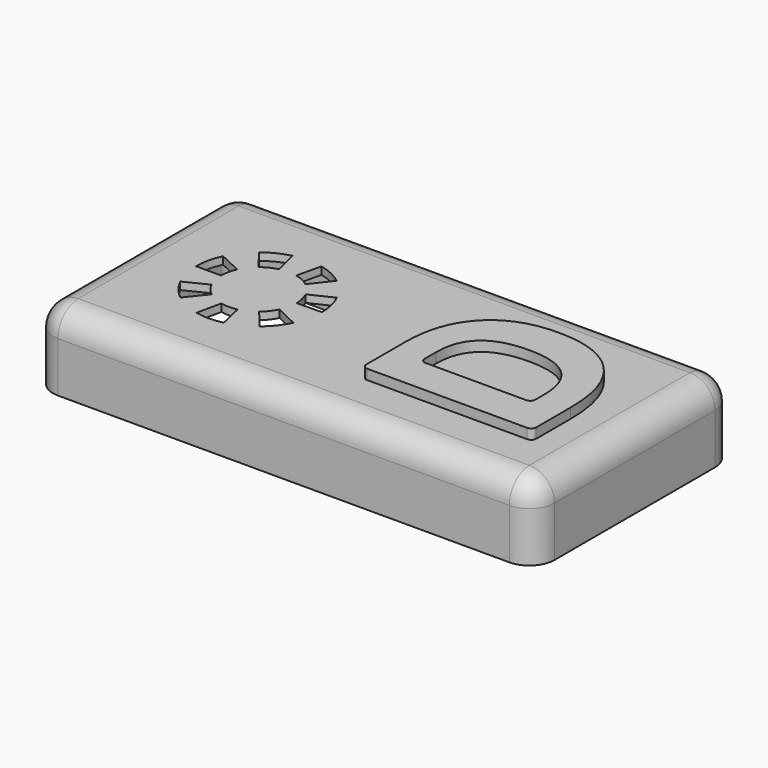
from build123d import *

# Parameters (mm, degrees)
F1_DEPTH     = 15
F2_R         = 5
F3_T         = -1.5
F5_DEPTH     = 1.5
F6_TEXT_SIZE = 47.5117315849
F7_DEPTH     = 2
F8_R         = 1


# Not quite as in the source:
# - Text() gives the source's letters only with a copy of the font that has no kerning and outlines rounded to 1/6400 em; it was checked with that copy


with BuildPart() as f1:
    # F0 (on Top) → F1 (new body)
    with BuildSketch(Plane.XY):
        with BuildLine():
            Line((45, 25), (-45, 25))
            ThreePointArc((-45, 25), (-48.5355339059, 23.5355339059), (-50, 20))
            Line((-50, 20), (-50, -20))
            ThreePointArc((-50, -20), (-48.5355339059, -23.5355339059), (-45, -25))
            Line((-45, -25), (45, -25))
            ThreePointArc((45, -25), (48.5355339059, -23.5355339059), (50, -20))
            Line((50, -20), (50, 20))
            ThreePointArc((50, 20), (48.5355339059, 23.5355339059), (45, 25))
        make_face()
    extrude(amount=F1_DEPTH)

    # F2
    f2_edges = [f1.edges().sort_by_distance(p)[0] for p in [
        (0, -25, 15),
    ]]
    fillet(f2_edges, radius=F2_R)

    # F3
    f3_openings = [f1.faces().sort_by_distance(p)[0] for p in [
        (0, 0, 0),
    ]]
    offset(amount=F3_T, openings=f3_openings)

    # F4 (on face) → F5 (cut, through all)
    with BuildSketch(Plane.XY.offset(15)):
        with BuildLine():
            ThreePointArc((-36.328847338, 5.2827282718), (-37.203700089, 2.7054951742), (-37.5, 0))
            Line((-37.5, 0), (-32.5, 0))
            ThreePointArc((-32.5, 0), (-32.3222200534, 1.6232971045), (-31.7973084028, 3.1696369631))
            Line((-31.7973084028, 3.1696369631), (-36.328847338, 5.2827282718))
        make_face()
        with BuildLine():
            ThreePointArc((-36.1936240582, -5.5635223055), (-34.7241238533, -7.8543882821), (-32.7936225232, -9.7728935309))
            Line((-32.7936225232, -9.7728935309), (-29.6761735139, -5.8637361185))
            ThreePointArc((-29.6761735139, -5.8637361185), (-30.834474312, -4.7126329692), (-31.7161744349, -3.3381133833))
            Line((-31.7161744349, -3.3381133833), (-36.1936240582, -5.5635223055))
        make_face()
        with BuildLine():
            ThreePointArc((-27.6293735543, -12.2203271115), (-24.9220840201, -12.4997571616), (-22.2184883255, -12.1865989023))
            Line((-22.2184883255, -12.1865989023), (-23.3310929953, -7.3119593414))
            ThreePointArc((-23.3310929953, -7.3119593414), (-24.9532504121, -7.499854297), (-26.5776241326, -7.3321962669))
            Line((-26.5776241326, -7.3321962669), (-27.6293735543, -12.2203271115))
        make_face()
        with BuildLine():
            ThreePointArc((-17.0851511346, -9.6749763533), (-15.178716509, -7.7325539499), (-13.7378891512, -5.423546739))
            Line((-13.7378891512, -5.423546739), (-18.2427334907, -3.2541280434))
            ThreePointArc((-18.2427334907, -3.2541280434), (-19.1072299054, -4.63953237), (-20.2510906807, -5.804985812))
            Line((-20.2510906807, -5.804985812), (-17.0851511346, -9.6749763533))
        make_face()
        with BuildLine():
            ThreePointArc((-12.500971344, 0.1558289324), (-12.8309757842, 2.8574201014), (-13.7378891512, 5.423546739))
            Line((-13.7378891512, 5.423546739), (-18.2427334907, 3.2541280434))
            ThreePointArc((-18.2427334907, 3.2541280434), (-17.6985854705, 1.7144520609), (-17.5005828064, 0.0934973595))
            Line((-17.5005828064, 0.0934973595), (-12.500971344, 0.1558289324))
        make_face()
        with BuildLine():
            ThreePointArc((-17.3288150651, 9.8692918538), (-19.6467584968, 11.2956985357), (-22.2184883255, 12.1865989023))
            Line((-22.2184883255, 12.1865989023), (-23.3310929953, 7.3119593414))
            ThreePointArc((-23.3310929953, 7.3119593414), (-21.7880550981, 6.7774191214), (-20.3972890391, 5.9215751123))
            Line((-20.3972890391, 5.9215751123), (-17.3288150651, 9.8692918538))
        make_face()
        with BuildLine():
            ThreePointArc((-27.9332175058, 12.1509767123), (-30.4936412476, 11.2280855823), (-32.7936225232, 9.7728935309))
            Line((-32.7936225232, 9.7728935309), (-29.6761735139, 5.8637361185))
            ThreePointArc((-29.6761735139, 5.8637361185), (-28.2961847485, 6.7368513494), (-26.7599305035, 7.2905860274))
            Line((-26.7599305035, 7.2905860274), (-27.9332175058, 12.1509767123))
        make_face()
    extrude(amount=-F5_DEPTH, mode=Mode.SUBTRACT)

    # F6 (on face) → F7 (join)
    with BuildSketch(Plane.XY.offset(15)):
        with Locations(Location((40.226809784, -17.6032576883), (0, 0, 90))):
            Text('D', F6_TEXT_SIZE, font='Open Sans', font_style=FontStyle.BOLD, text_align=(TextAlign.LEFT, TextAlign.BOTTOM))
    extrude(amount=F7_DEPTH)

    # F8
    f8_edges = [f1.edges().sort_by_distance(p)[0] for p in [
        (6.307888, -13.334626, 16),
        (40.22681, -13.334626, 16),
        (12.202312, -6.141052, 16),
        (34.287843, -6.141052, 16),
    ]]
    fillet(f8_edges, radius=F8_R)


solid = f1.part
